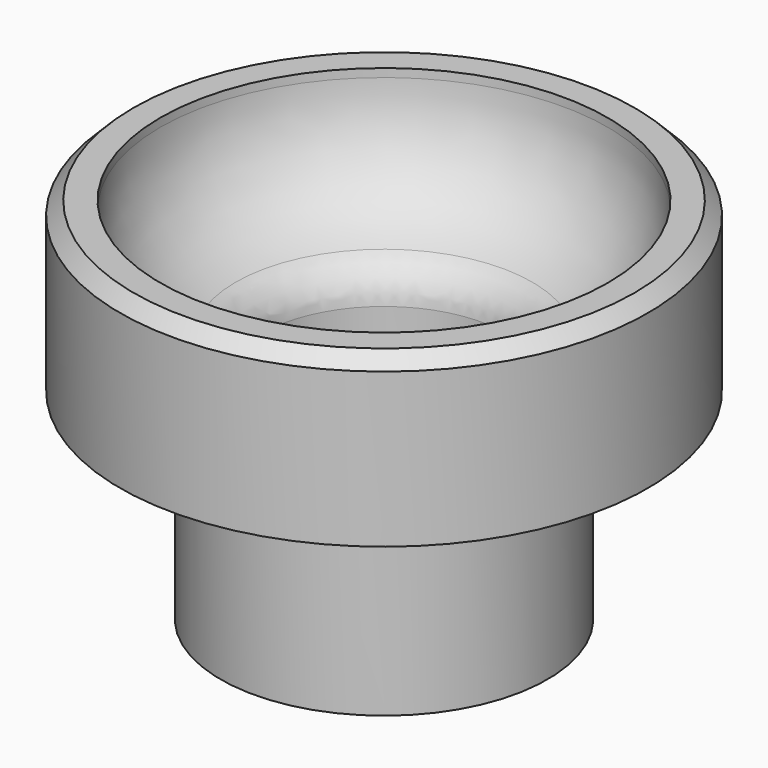
from build123d import *

# Parameters (mm, degrees)
F3_R    = 1.2
F4_SIZE = 0.4


# Not quite as in the source:
# - a fillet or chamfer that OpenCascade refuses, or shapes differently, is made with other operations: its cross-section is extruded or revolved along the edge and cut away or added


with BuildPart() as f1:
    # F0 (on Front) → F1 (revolve)
    with BuildSketch(Plane.XZ):
        Polygon((-4.875, 6), (-4.875, 0), (-3.675, 0), (-3.675, 7.2), (-6.675, 7.2), (-6.675, 11), (-7.875, 11), (-7.875, 6), align=None)
    revolve(axis=Axis((0, 0, 5.5), (0, 0, 1)))

    # F2: fillet of radius 3.6 on 1 edges, made by hand

    # F2_s1 → F2_t2 (revolve)
    with BuildSketch(Plane.XZ):
        with BuildLine():
            ThreePointArc((-3.675, 7.2), (-5.824545417, 8.4258578621), (-6.675, 10.7496478699))
            Line((-6.675, 10.7496478699), (-6.675, 7.2))
            Line((-6.675, 7.2), (-3.675, 7.2))
        make_face()
    revolve(axis=Axis((0, 0, 7.2), (0, 0, 1)))

    # F3
    f3_edges = [f1.edges().sort_by_distance(p)[0] for p in [
        (3.675, 0, 7.2),
    ]]
    fillet(f3_edges, radius=F3_R)

    # F4
    f4_edges = [f1.edges().sort_by_distance(p)[0] for p in [
        (7.875, 0, 11),
        (3.675, 0, 0),
    ]]
    chamfer(f4_edges, length=F4_SIZE)


solid = f1.part
